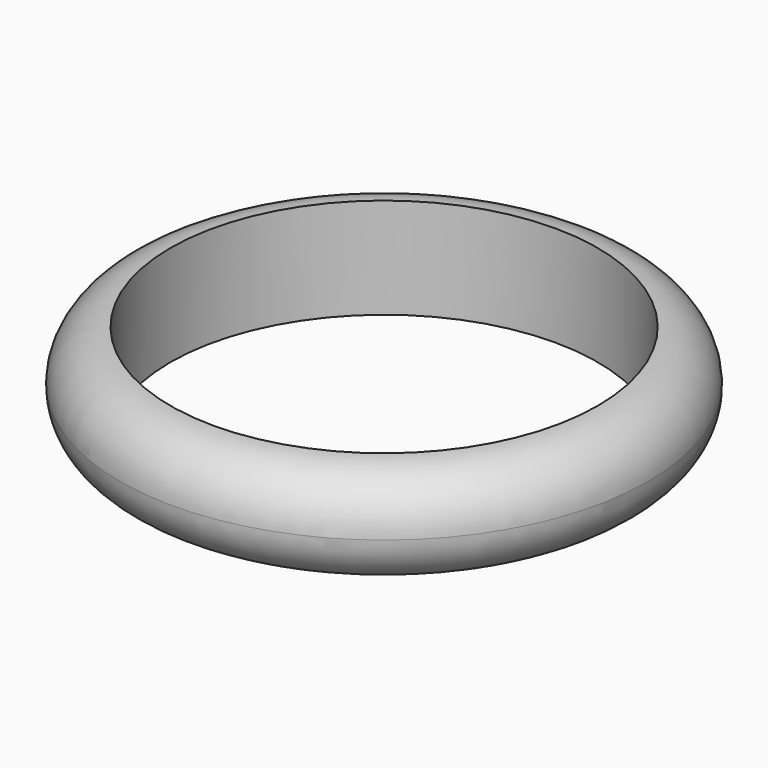
from build123d import *

# Parameters (mm, degrees)
F0_R     = 10.5
F0_R_2   = 8.5
F1_DEPTH = 4
F2_R     = 1.99999


# Not quite as in the source:
# - a fillet or chamfer is up to 0.001 mm smaller than in the source, because OpenCascade refuses the exact size


with BuildPart() as f1:
    # F0 (on Top) → F1 (new body)
    with BuildSketch(Plane.XY):
        Circle(F0_R)
        Circle(F0_R_2, mode=Mode.SUBTRACT)
    extrude(amount=F1_DEPTH)

    # F2 (radius 2 in the source; OpenCascade refuses exactly that, so slightly less here)
    f2_edges = [f1.edges().sort_by_distance(p)[0] for p in [
        (-10.5, 0, 4),
        (-10.5, 0, 0),
    ]]
    fillet(f2_edges, radius=F2_R)


solid = f1.part
